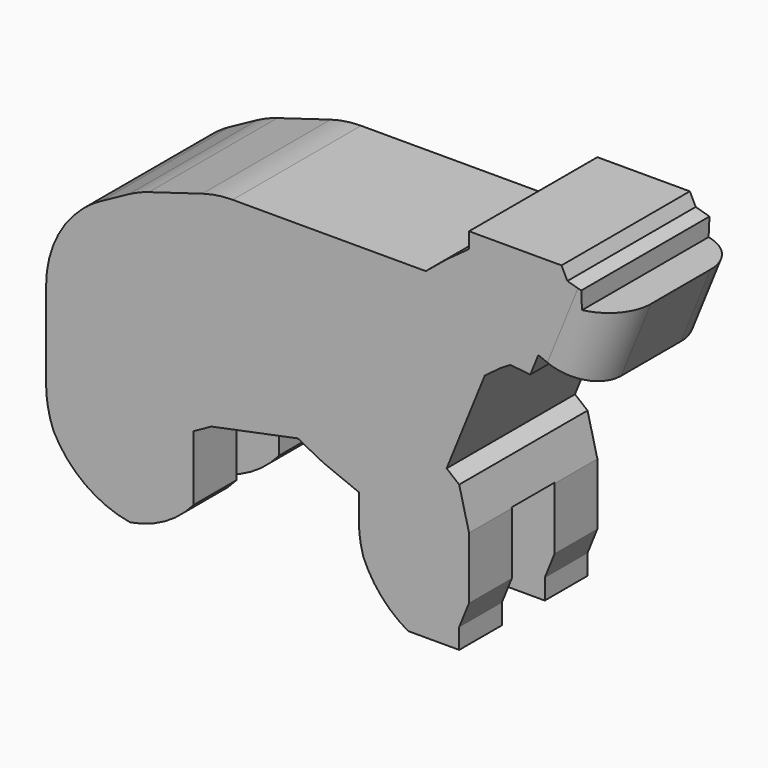
from build123d import *

# Parameters (mm, degrees)
F1_DEPTH     = 19.05
F2_T1_DEPTH  = 28.2300180496
F2_T3_DEPTH  = 25.482580603
F2_T5_DEPTH  = 25.9366089247
F2_T7_DEPTH  = 47.5485210799
F2_T9_DEPTH  = 32.7314977927
F2_T11_DEPTH = 59.1455336843
F2_T13_DEPTH = 52.8213628452
F2_T15_DEPTH = 21.9875710363
F2_T17_DEPTH = 46.4468482438
F2_T19_DEPTH = 29.758572197
F3_R         = 5.08
F5_W         = 6.35
F5_H         = 12.7
F6_DEPTH     = 303.0582275594


# Not quite as in the source:
# - a fillet or chamfer that OpenCascade refuses, or shapes differently, is made with other operations: its cross-section is extruded or revolved along the edge and cut away or added


with BuildPart() as f1:
    # F0 (on Front) → F1 (new body)
    with BuildSketch(Plane.XZ):
        Polygon((-45.0859302655, 0.4672128707), (-34.340060316, 0.4672128707), (-31.5367905423, 4.9057230353), (-31.5367905423, 9.1106286272), (-31.5367905423, 12.6147158444), (-29.4343372807, 13.7827442959), (-19.1556811333, 15.8851970918), (-16.2193404098, 14.3601642462), (-11.9138995651, 12.6147158444), (-11.9138995651, 9.1106286272), (-11.9138995651, 7.4753854424), (-9.811447002, 1.5152803213), (-6.0737542808, 0), (0, 0), (0, 2.3983575983), (1.1680293828, 5.2794977153), (1.1680293828, 9.1106286272), (1.1680293828, 12.6147158444), (0, 17.2868324444), (-1.4916199837, 18.4976548306), (3.0368734151, 29.6679423191), (4.9057211727, 31.0695767403), (6.0737496242, 31.770395115), (8.4476916948, 31.5367886797), (9.3986034807, 33.8823718767), (12.8483185545, 32.4838392109), (15.1843773201, 31.5367886797), (18.6884636059, 40.1802044362), (14.483560808, 40.1802044362), (14.483560808, 42.2826576978), (12.8483185545, 42.7498687059), (12.1475020424, 44.1515035927), (8.1762028858, 44.1515035927), (5.3729321808, 44.1515035927), (1.1680293828, 44.1515035927), (1.1680293828, 42.2826576978), (-1.4016367495, 40.4138118029), (-3.9712996222, 38.3113585413), (-14.7171695717, 38.3113585413), (-22.192556411, 38.3113585413), (-28.7335207686, 38.3113585413), (-38.0777539685, 35.5080878362), (-43.684293516, 32.4712125584), (-49.0572275594, 27.7990954928), (-49.0572275594, 14.9507736787), (-49.0572275594, 9.1106286272), align=None)
    extrude(amount=F1_DEPTH)

    # F2: fillet of radius 12.5094889948 on 10 edges, made by hand

    # F2_s2 → F2_t1 (cut)
    with BuildSketch(Plane.XZ.offset(-4.5900090248)):
        with BuildLine():
            ThreePointArc((-30.4920932473, 37.7837866574), (-28.7140598467, 38.1787628389), (-26.8975171587, 38.3113585413))
            Line((-26.8975171587, 38.3113585413), (-28.7335207686, 38.3113585413))
            Line((-28.7335207686, 38.3113585413), (-30.4920932473, 37.7837866574))
        make_face()
    extrude(amount=F2_T1_DEPTH, mode=Mode.SUBTRACT)

    # F2_s4 → F2_t3 (cut)
    with BuildSketch(Plane.XZ.offset(-3.2162903015)):
        with BuildLine():
            ThreePointArc((-39.2089772844, 34.8953419361), (-38.0524286269, 35.4471609705), (-36.8454950389, 35.8777656133))
            Line((-36.8454950389, 35.8777656133), (-38.0777539685, 35.5080878362))
            Line((-38.0777539685, 35.5080878362), (-39.2089772844, 34.8953419361))
        make_face()
    extrude(amount=F2_T3_DEPTH, mode=Mode.SUBTRACT)

    # F2_s6 → F2_t5 (cut)
    with BuildSketch(Plane.XZ.offset(-3.4433044624)):
        with BuildLine():
            ThreePointArc((-42.4732255071, 33.1272076629), (-43.6412308258, 32.4090824128), (-44.7236280922, 31.5674432638))
            Line((-44.7236280922, 31.5674432638), (-43.684293516, 32.4712125584))
            Line((-43.684293516, 32.4712125584), (-42.4732255071, 33.1272076629))
        make_face()
    extrude(amount=F2_T5_DEPTH, mode=Mode.SUBTRACT)

    # F2_s8 → F2_t7 (cut)
    with BuildSketch(Plane.XZ.offset(-14.2492605399)):
        with BuildLine():
            ThreePointArc((-49.0572275594, 22.0993912768), (-47.9313005389, 27.2860888474), (-44.7561994839, 31.5391203114))
            Line((-44.7561994839, 31.5391203114), (-49.0572275594, 27.7990954928))
            Line((-49.0572275594, 27.7990954928), (-49.0572275594, 22.0993912768))
        make_face()
    extrude(amount=F2_T7_DEPTH, mode=Mode.SUBTRACT)

    # F2_s10 → F2_t9 (cut)
    with BuildSketch(Plane.XZ.offset(-6.8407488963)):
        with BuildLine():
            ThreePointArc((-49.0572275594, 11.8469281858), (-48.7682894076, 9.1738303565), (-47.9148224607, 6.6242163797))
            Line((-47.9148224607, 6.6242163797), (-49.0572275594, 9.1106286272))
            Line((-49.0572275594, 9.1106286272), (-49.0572275594, 11.8469281858))
        make_face()
    extrude(amount=F2_T9_DEPTH, mode=Mode.SUBTRACT)

    # F2_s12 → F2_t11 (cut)
    with BuildSketch(Plane.XZ.offset(-20.0477668422)):
        with BuildLine():
            ThreePointArc((-37.0668235286, 0.4672128707), (-43.8178922977, 2.4453018928), (-48.4339074248, 7.7539900595))
            Line((-48.4339074248, 7.7539900595), (-45.0859302655, 0.4672128707))
            Line((-45.0859302655, 0.4672128707), (-37.0668235286, 0.4672128707))
        make_face()
    extrude(amount=F2_T11_DEPTH, mode=Mode.SUBTRACT)

    # F2_s14 → F2_t13 (cut)
    with BuildSketch(Plane.XZ.offset(-16.8856814226)):
        with BuildLine():
            ThreePointArc((-31.5367905423, 4.9057230353), (-35.825391148, 1.6309728064), (-41.0943328851, 0.4672128707))
            Line((-41.0943328851, 0.4672128707), (-34.340060316, 0.4672128707))
            Line((-34.340060316, 0.4672128707), (-31.5367905423, 4.9057230353))
        make_face()
    extrude(amount=F2_T13_DEPTH, mode=Mode.SUBTRACT)

    # F2_s16 → F2_t15 (cut)
    with BuildSketch(Plane.XZ.offset(-1.4687855182)):
        with BuildLine():
            ThreePointArc((-15.6748678973, 14.139432221), (-16.2135660804, 14.3726858024), (-16.7407283206, 14.6309549221))
            Line((-16.7407283206, 14.6309549221), (-16.2193404098, 14.3601642462))
            Line((-16.2193404098, 14.3601642462), (-15.6748678973, 14.139432221))
        make_face()
    extrude(amount=F2_T15_DEPTH, mode=Mode.SUBTRACT)

    # F2_s18 → F2_t17 (cut)
    with BuildSketch(Plane.XZ.offset(-13.6984241219)):
        with BuildLine():
            ThreePointArc((-6.0737542808, 0), (-9.4531651589, 2.8427255588), (-11.6342326331, 6.6825759671))
            Line((-11.6342326331, 6.6825759671), (-9.811447002, 1.5152803213))
            Line((-9.811447002, 1.5152803213), (-6.0737542808, 0))
        make_face()
    extrude(amount=F2_T17_DEPTH, mode=Mode.SUBTRACT)

    # F2_s20 → F2_t19 (cut)
    with BuildSketch(Plane.XZ.offset(-5.3542860985)):
        with BuildLine():
            ThreePointArc((-11.2014295993, 5.4556509826), (-11.7344956192, 7.5061006875), (-11.9138995651, 9.6170998818))
            Line((-11.9138995651, 9.6170998818), (-11.9138995651, 7.4753854424))
            Line((-11.9138995651, 7.4753854424), (-11.2014295993, 5.4556509826))
        make_face()
    extrude(amount=F2_T19_DEPTH, mode=Mode.SUBTRACT)

    # F3
    f3_edges = [f1.edges().sort_by_distance(p)[0] for p in [
        (16.93642, 0, 35.858497),
        (16.93642, -19.05, 35.858497),
    ]]
    fillet(f3_edges, radius=F3_R)

    # F5 (on offset) → F6 (cut, through all)
    with BuildSketch(Plane.YZ.offset(254)):
        with Locations((-9.525, 6.35)):
            Rectangle(F5_W, F5_H)
    extrude(amount=-F6_DEPTH, mode=Mode.SUBTRACT)


solid = f1.part
